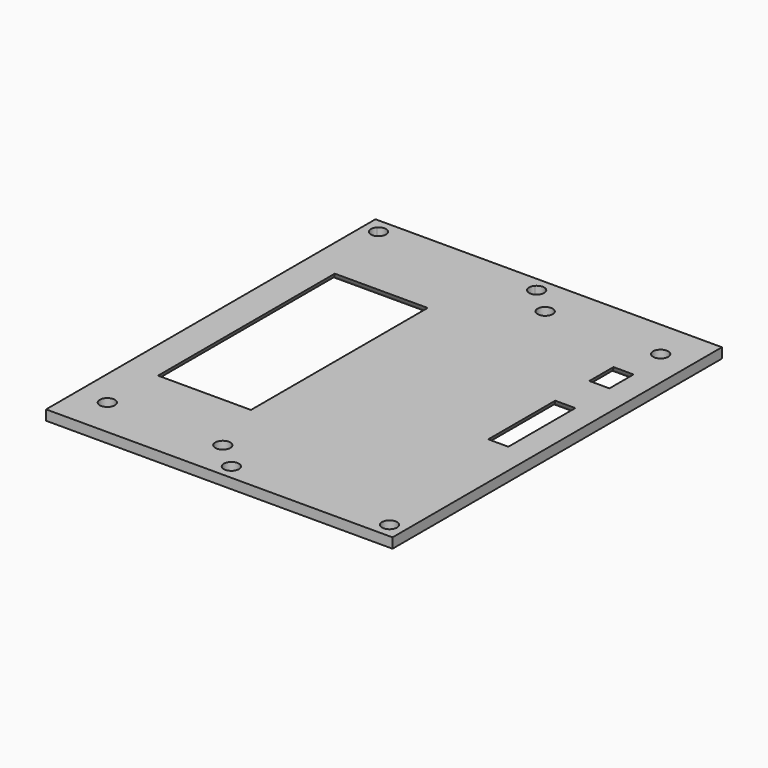
from build123d import *

# Parameters (mm, degrees)
F0_R          = 1.5
F0_W          = 18.5
F0_H          = 44
F0_W_2        = 4
F0_H_2        = 16.6644380502
F0_H_3        = 6
F0_W_3        = 4.7
F0_H_4        = 2
F0_W_4        = 13
F0_W_5        = 2.3
F0_W_6        = 1.5
F0_W_7        = 9
F0_W_8        = 11
F1_DEPTH      = 2
F2_T1_DEPTH   = 16.6644380502
F2_T3_DEPTH   = 4
F2_T5_DEPTH   = 6
F2_T7_DEPTH   = 44
F2_T9_DEPTH   = 18.5
F2_T15_DEPTH  = 11.0710678119
F2_T19_DEPTH  = 23.7355058621
F2_T26_DEPTH  = 11.0710678119
F2_T30_DEPTH  = 23.7355058621
F2_T37_DEPTH  = 23.7355058621
F2_T41_DEPTH  = 11.0710678119
F2_T49_DEPTH  = 11.0710678119
F2_T54_DEPTH  = 23.7355058621
F2_T61_DEPTH  = 13.0710678119
F2_T65_DEPTH  = 11.0710678119
F2_T73_DEPTH  = 13.0710678119
F2_T77_DEPTH  = 11.0710678119
F2_T84_DEPTH  = 11.0710678119
F2_T89_DEPTH  = 13.0710678119
F2_S91_R      = 1.5
F2_T92_DEPTH  = 8
F2_T98_DEPTH  = 13.0710678119
F2_T102_DEPTH = 11.0710678119
F2_T109_DEPTH = 25.5710678119
F2_T113_DEPTH = 51.0710678119
F2_T120_DEPTH = 51.0710678119
F2_T124_DEPTH = 25.5710678119
F2_T131_DEPTH = 51.0710678119
F2_T135_DEPTH = 25.5710678119
F2_T143_DEPTH = 51.0710678119
F2_T147_DEPTH = 25.5710678119


# Not quite as in the source:
# - a fillet or chamfer that OpenCascade refuses, or shapes differently, is made with other operations: its cross-section is extruded or revolved along the edge and cut away or added


with BuildPart() as f1:
    # F0 (on Top) → F1 (new body)
    with BuildSketch(Plane.XY):
        with BuildLine():
            Line((12.5, -41), (34.5, -41))
            Line((34.5, -41), (34.5, 39))
            Line((34.5, 39), (28.5, 39))
            Line((28.5, 39), (25.5, 39))
            Line((25.5, 39), (20.8, 39))
            Line((20.8, 39), (7.8, 39))
            Line((7.8, 39), (5.5, 39))
            Line((5.5, 39), (1.1180339887, 39))
            ThreePointArc((1.1180339887, 39), (1.4012585384, 38.5352331347), (1.5, 38))
            ThreePointArc((1.5, 38), (-0.5352331347, 36.5987414616), (-1.1180339887, 39))
            Line((-1.1180339887, 39), (-5.5, 39))
            Line((-5.5, 39), (-14.5, 39))
            Line((-14.5, 39), (-25.5, 39))
            Line((-25.5, 39), (-27, 39))
            Line((-27, 39), (-28.5, 39))
            Line((-28.5, 39), (-30.3819660113, 39))
            ThreePointArc((-30.3819660113, 39), (-30.0987414616, 38.5352331347), (-30, 38))
            ThreePointArc((-30, 38), (-32.0352331347, 36.5987414616), (-32.6180339887, 39))
            Line((-32.6180339887, 39), (-34.5, 39))
            Line((-34.5, 39), (-34.5, -41))
            Line((-34.5, -41), (-12.5, -41))
            Line((-12.5, -41), (-10.5, -41))
            Line((-10.5, -41), (10.5, -41))
            Line((10.5, -41), (12.5, -41))
        make_face()
        with Locations((-28.5, -33.25)):
            Circle(F0_R, mode=Mode.SUBTRACT)
        with Locations((-5.5, -33.25)):
            Circle(F0_R, mode=Mode.SUBTRACT)
        with Locations((0, -38)):
            Circle(F0_R, mode=Mode.SUBTRACT)
        with Locations((31.5, -38)):
            Circle(F0_R, mode=Mode.SUBTRACT)
        with Locations((-18.75, 0.75)):
            Rectangle(F0_W, F0_H, mode=Mode.SUBTRACT)
        with Locations((-28.5, 33.25)):
            Circle(F0_R, mode=Mode.SUBTRACT)
        with Locations((-5.5, 33.25)):
            Circle(F0_R, mode=Mode.SUBTRACT)
        with Locations((27.5, 2.4177809749)):
            Rectangle(F0_W_2, F0_H_2, mode=Mode.SUBTRACT)
        with Locations((5.5, 33.25)):
            Circle(F0_R, mode=Mode.SUBTRACT)
        with Locations((27.5, 22.25)):
            Rectangle(F0_W_2, F0_H_3, mode=Mode.SUBTRACT)
        with Locations((28.5, 33.25)):
            Circle(F0_R, mode=Mode.SUBTRACT)
        Polygon((28.5, 39), (34.5, 39), (34.5, 41), (28, 41), (25.5, 41), (25.5, 39), align=None)
        with Locations((23.15, 40)):
            Rectangle(F0_W_3, F0_H_4)
        with Locations((14.3, 40)):
            Rectangle(F0_W_4, F0_H_4)
        with Locations((6.65, 40)):
            Rectangle(F0_W_5, F0_H_4)
        with BuildLine():
            Line((-34.5, 41), (-34.5, 39))
            Line((-34.5, 39), (-32.6180339887, 39))
            ThreePointArc((-32.6180339887, 39), (-31.5, 39.5), (-30.3819660113, 39))
            Line((-30.3819660113, 39), (-28.5, 39))
            Line((-28.5, 39), (-27, 39))
            Line((-27, 39), (-27, 41))
            Line((-27, 41), (-34.5, 41))
        make_face()
        with BuildLine():
            Line((1.1180339887, 39), (5.5, 39))
            Line((5.5, 39), (5.5, 41))
            Line((5.5, 41), (-5.5, 41))
            Line((-5.5, 41), (-5.5, 39))
            Line((-5.5, 39), (-1.1180339887, 39))
            ThreePointArc((-1.1180339887, 39), (0, 39.5), (1.1180339887, 39))
        make_face()
        with Locations((-26.25, 40)):
            Rectangle(F0_W_6, F0_H_4)
        with Locations((-10, 40)):
            Rectangle(F0_W_7, F0_H_4)
        with Locations((-20, 40)):
            Rectangle(F0_W_8, F0_H_4)
        with Locations((-28.5, 33.25)):
            Circle(F0_R)
        with Locations((-5.5, 33.25)):
            Circle(F0_R)
    extrude(amount=F1_DEPTH)

    # F2: fillet of radius 3 on 12 edges, made by hand

    # F2_s2 → F2_t1 (cut)
    with BuildSketch(Plane.XZ.offset(-10.75)):
        with BuildLine():
            ThreePointArc((25.5, 2), (24.4036236828, 0.5505102572), (22.6715728753, 0))
            Line((22.6715728753, 0), (25.5, 0))
            Line((25.5, 0), (25.5, 2))
        make_face()
        with BuildLine():
            ThreePointArc((29.5, 2), (30.5963763172, 0.5505102572), (32.3284271247, 0))
            Line((32.3284271247, 0), (29.5, 0))
            Line((29.5, 0), (29.5, 2))
        make_face()
    extrude(amount=F2_T1_DEPTH, mode=Mode.SUBTRACT)

    # F2_s4 → F2_t3 (cut)
    with BuildSketch(Plane.YZ.offset(25.5)):
        with BuildLine():
            ThreePointArc((-5.9144380502, 2), (-7.0108143674, 0.5505102572), (-8.742865175, 0))
            Line((-8.742865175, 0), (-5.9144380502, 0))
            Line((-5.9144380502, 0), (-5.9144380502, 2))
        make_face()
        with BuildLine():
            ThreePointArc((10.75, 2), (11.8463763172, 0.5505102572), (13.5784271247, 0))
            Line((13.5784271247, 0), (10.75, 0))
            Line((10.75, 0), (10.75, 2))
        make_face()
        with BuildLine():
            ThreePointArc((19.25, 2), (18.1536236828, 0.5505102572), (16.4215728753, 0))
            Line((16.4215728753, 0), (19.25, 0))
            Line((19.25, 0), (19.25, 2))
        make_face()
        with BuildLine():
            ThreePointArc((25.25, 2), (26.3463763172, 0.5505102572), (28.0784271247, 0))
            Line((28.0784271247, 0), (25.25, 0))
            Line((25.25, 0), (25.25, 2))
        make_face()
    extrude(amount=F2_T3_DEPTH, mode=Mode.SUBTRACT)

    # F2_s6 → F2_t5 (cut)
    with BuildSketch(Plane.XZ.offset(-25.25)):
        with BuildLine():
            ThreePointArc((29.5, 2), (30.5963763172, 0.5505102572), (32.3284271247, 0))
            Line((32.3284271247, 0), (29.5, 0))
            Line((29.5, 0), (29.5, 2))
        make_face()
        with BuildLine():
            ThreePointArc((25.5, 2), (24.4036236828, 0.5505102572), (22.6715728753, 0))
            Line((22.6715728753, 0), (25.5, 0))
            Line((25.5, 0), (25.5, 2))
        make_face()
    extrude(amount=F2_T5_DEPTH, mode=Mode.SUBTRACT)

    # F2_s8 → F2_t7 (cut)
    with BuildSketch(Plane.XZ.offset(-22.75)):
        with BuildLine():
            ThreePointArc((-9.5, 2), (-8.4036236828, 0.5505102572), (-6.6715728753, 0))
            Line((-6.6715728753, 0), (-9.5, 0))
            Line((-9.5, 0), (-9.5, 2))
        make_face()
        with BuildLine():
            ThreePointArc((-28, 2), (-29.0963763172, 0.5505102572), (-30.8284271247, 0))
            Line((-30.8284271247, 0), (-28, 0))
            Line((-28, 0), (-28, 2))
        make_face()
    extrude(amount=F2_T7_DEPTH, mode=Mode.SUBTRACT)

    # F2_s10 → F2_t9 (cut)
    with BuildSketch(Plane.YZ.offset(-28)):
        with BuildLine():
            ThreePointArc((-21.25, 2), (-22.3463763172, 0.5505102572), (-24.0784271247, 0))
            Line((-24.0784271247, 0), (-21.25, 0))
            Line((-21.25, 0), (-21.25, 2))
        make_face()
        with BuildLine():
            ThreePointArc((22.75, 2), (23.8463763172, 0.5505102572), (25.5784271247, 0))
            Line((25.5784271247, 0), (22.75, 0))
            Line((22.75, 0), (22.75, 2))
        make_face()
    extrude(amount=F2_T9_DEPTH, mode=Mode.SUBTRACT)


with BuildPart() as f2_tool13:
    # F2_s14 → F2_t15 (new body)
    with BuildSketch(Plane.YZ.offset(29.5)):
        with BuildLine():
            ThreePointArc((-5.9144380502, 2), (-7.0108143674, 0.5505102572), (-8.742865175, 0))
            Line((-8.742865175, 0), (-5.9144380502, 0))
            Line((-5.9144380502, 0), (-5.9144380502, 2))
        make_face()
    extrude(amount=-F2_T15_DEPTH)

    split(bisect_by=Plane.YZ.offset(25.5), keep=Keep.BOTTOM)


with BuildPart() as f2_tool17:
    # F2_s18 → F2_t19 (new body)
    with BuildSketch(Plane.XZ.offset(12.9855058621)):
        with BuildLine():
            ThreePointArc((25.5, 2), (24.4036236828, 0.5505102572), (22.6715728753, 0))
            Line((22.6715728753, 0), (25.5, 0))
            Line((25.5, 0), (25.5, 2))
        make_face()
    extrude(amount=-F2_T19_DEPTH)

    split(bisect_by=Plane.XZ.offset(5.9144380502), keep=Keep.TOP)


with BuildPart() as f2_tool13_1:
    add(f2_tool13.part)

    # F2_t21: intersect F2_tool17
    add(f2_tool17.part, mode=Mode.INTERSECT)


with BuildPart() as f1_1:
    add(f1.part)

    # F2_t11: cut F2_tool13
    add(f2_tool13_1.part, mode=Mode.SUBTRACT)


with BuildPart() as f2_tool24:
    # F2_s25 → F2_t26 (new body)
    with BuildSketch(Plane.YZ.offset(18.4289321881)):
        with BuildLine():
            ThreePointArc((10.75, 2), (11.8463763172, 0.5505102572), (13.5784271247, 0))
            Line((13.5784271247, 0), (10.75, 0))
            Line((10.75, 0), (10.75, 2))
        make_face()
    extrude(amount=F2_T26_DEPTH)

    split(bisect_by=Plane.YZ.offset(25.5), keep=Keep.BOTTOM)


with BuildPart() as f2_tool28:
    # F2_s29 → F2_t30 (new body)
    with BuildSketch(Plane.XZ.offset(5.9144380502)):
        with BuildLine():
            ThreePointArc((25.5, 2), (24.4036236828, 0.5505102572), (22.6715728753, 0))
            Line((22.6715728753, 0), (25.5, 0))
            Line((25.5, 0), (25.5, 2))
        make_face()
    extrude(amount=-F2_T30_DEPTH)

    split(bisect_by=Plane.XZ.offset(-10.75), keep=Keep.BOTTOM)


with BuildPart() as f2_tool24_1:
    add(f2_tool24.part)

    # F2_t32: intersect F2_tool28
    add(f2_tool28.part, mode=Mode.INTERSECT)


with BuildPart() as f1_2:
    add(f1_1.part)

    # F2_t22: cut F2_tool24
    add(f2_tool24_1.part, mode=Mode.SUBTRACT)


with BuildPart() as f2_tool35:
    # F2_s36 → F2_t37 (new body)
    with BuildSketch(Plane.XZ.offset(-10.75)):
        with BuildLine():
            ThreePointArc((29.5, 2), (30.5963763172, 0.5505102572), (32.3284271247, 0))
            Line((32.3284271247, 0), (29.5, 0))
            Line((29.5, 0), (29.5, 2))
        make_face()
    extrude(amount=F2_T37_DEPTH)

    split(bisect_by=Plane.XZ.offset(5.9144380502), keep=Keep.TOP)


with BuildPart() as f2_tool39:
    # F2_s40 → F2_t41 (new body)
    with BuildSketch(Plane.YZ.offset(36.5710678119)):
        with BuildLine():
            ThreePointArc((-5.9144380502, 2), (-7.0108143674, 0.5505102572), (-8.742865175, 0))
            Line((-8.742865175, 0), (-5.9144380502, 0))
            Line((-5.9144380502, 0), (-5.9144380502, 2))
        make_face()
    extrude(amount=-F2_T41_DEPTH)

    split(bisect_by=Plane.YZ.offset(34.5), keep=Keep.BOTTOM)

    split(bisect_by=Plane.YZ.offset(29.5), keep=Keep.TOP)


with BuildPart() as f2_tool35_1:
    add(f2_tool35.part)

    # F2_t44: intersect F2_tool39
    add(f2_tool39.part, mode=Mode.INTERSECT)


with BuildPart() as f1_3:
    add(f1_2.part)

    # F2_t33: cut F2_tool35
    add(f2_tool35_1.part, mode=Mode.SUBTRACT)


with BuildPart() as f2_tool47:
    # F2_s48 → F2_t49 (new body)
    with BuildSketch(Plane.YZ.offset(25.5)):
        with BuildLine():
            ThreePointArc((10.75, 2), (11.8463763172, 0.5505102572), (13.5784271247, 0))
            Line((13.5784271247, 0), (10.75, 0))
            Line((10.75, 0), (10.75, 2))
        make_face()
    extrude(amount=F2_T49_DEPTH)

    split(bisect_by=Plane.YZ.offset(34.5), keep=Keep.BOTTOM)

    split(bisect_by=Plane.YZ.offset(29.5), keep=Keep.TOP)


with BuildPart() as f2_tool52:
    # F2_s53 → F2_t54 (new body)
    with BuildSketch(Plane.XZ.offset(-17.8210678119)):
        with BuildLine():
            ThreePointArc((29.5, 2), (30.5963763172, 0.5505102572), (32.3284271247, 0))
            Line((32.3284271247, 0), (29.5, 0))
            Line((29.5, 0), (29.5, 2))
        make_face()
    extrude(amount=F2_T54_DEPTH)

    split(bisect_by=Plane.XZ.offset(-10.75), keep=Keep.BOTTOM)


with BuildPart() as f2_tool47_1:
    add(f2_tool47.part)

    # F2_t56: intersect F2_tool52
    add(f2_tool52.part, mode=Mode.INTERSECT)


with BuildPart() as f1_4:
    add(f1_3.part)

    # F2_t45: cut F2_tool47
    add(f2_tool47_1.part, mode=Mode.SUBTRACT)


with BuildPart() as f2_tool59:
    # F2_s60 → F2_t61 (new body)
    with BuildSketch(Plane.XZ.offset(-25.25)):
        with BuildLine():
            ThreePointArc((29.5, 2), (30.5963763172, 0.5505102572), (32.3284271247, 0))
            Line((32.3284271247, 0), (29.5, 0))
            Line((29.5, 0), (29.5, 2))
        make_face()
    extrude(amount=F2_T61_DEPTH)

    split(bisect_by=Plane.XZ.offset(-19.25), keep=Keep.TOP)


with BuildPart() as f2_tool63:
    # F2_s64 → F2_t65 (new body)
    with BuildSketch(Plane.YZ.offset(36.5710678119)):
        with BuildLine():
            ThreePointArc((19.25, 2), (18.1536236828, 0.5505102572), (16.4215728753, 0))
            Line((16.4215728753, 0), (19.25, 0))
            Line((19.25, 0), (19.25, 2))
        make_face()
    extrude(amount=-F2_T65_DEPTH)

    split(bisect_by=Plane.YZ.offset(34.5), keep=Keep.BOTTOM)

    split(bisect_by=Plane.YZ.offset(29.5), keep=Keep.TOP)


with BuildPart() as f2_tool59_1:
    add(f2_tool59.part)

    # F2_t68: intersect F2_tool63
    add(f2_tool63.part, mode=Mode.INTERSECT)


with BuildPart() as f1_5:
    add(f1_4.part)

    # F2_t57: cut F2_tool59
    add(f2_tool59_1.part, mode=Mode.SUBTRACT)


with BuildPart() as f2_tool71:
    # F2_s72 → F2_t73 (new body)
    with BuildSketch(Plane.XZ.offset(-12.1789321881)):
        with BuildLine():
            ThreePointArc((25.5, 2), (24.4036236828, 0.5505102572), (22.6715728753, 0))
            Line((22.6715728753, 0), (25.5, 0))
            Line((25.5, 0), (25.5, 2))
        make_face()
    extrude(amount=-F2_T73_DEPTH)

    split(bisect_by=Plane.XZ.offset(-19.25), keep=Keep.TOP)


with BuildPart() as f2_tool75:
    # F2_s76 → F2_t77 (new body)
    with BuildSketch(Plane.YZ.offset(29.5)):
        with BuildLine():
            ThreePointArc((19.25, 2), (18.1536236828, 0.5505102572), (16.4215728753, 0))
            Line((16.4215728753, 0), (19.25, 0))
            Line((19.25, 0), (19.25, 2))
        make_face()
    extrude(amount=-F2_T77_DEPTH)

    split(bisect_by=Plane.YZ.offset(25.5), keep=Keep.BOTTOM)


with BuildPart() as f2_tool71_1:
    add(f2_tool71.part)

    # F2_t79: intersect F2_tool75
    add(f2_tool75.part, mode=Mode.INTERSECT)


with BuildPart() as f1_6:
    add(f1_5.part)

    # F2_t69: cut F2_tool71
    add(f2_tool71_1.part, mode=Mode.SUBTRACT)


with BuildPart() as f2_tool82:
    # F2_s83 → F2_t84 (new body)
    with BuildSketch(Plane.YZ.offset(25.5)):
        with BuildLine():
            ThreePointArc((25.25, 2), (26.3463763172, 0.5505102572), (28.0784271247, 0))
            Line((28.0784271247, 0), (25.25, 0))
            Line((25.25, 0), (25.25, 2))
        make_face()
    extrude(amount=F2_T84_DEPTH)

    split(bisect_by=Plane.YZ.offset(34.5), keep=Keep.BOTTOM)

    split(bisect_by=Plane.YZ.offset(29.5), keep=Keep.TOP)


with BuildPart() as f2_tool87:
    # F2_s88 → F2_t89 (new body)
    with BuildSketch(Plane.XZ.offset(-32.3210678119)):
        with BuildLine():
            ThreePointArc((29.5, 2), (30.5963763172, 0.5505102572), (32.3284271247, 0))
            Line((32.3284271247, 0), (29.5, 0))
            Line((29.5, 0), (29.5, 2))
        make_face()
    extrude(amount=F2_T89_DEPTH)

    split(bisect_by=Plane.XZ.offset(-25.25), keep=Keep.BOTTOM)

    # F2_s91 → F2_t92 (cut, symmetric)
    with BuildSketch(Plane.XY.offset(1)):
        with Locations((28.5, 33.25)):
            Circle(F2_S91_R)
    extrude(amount=F2_T92_DEPTH, both=True, mode=Mode.SUBTRACT)


with BuildPart() as f2_tool82_1:
    add(f2_tool82.part)

    # F2_t93: intersect F2_tool87
    add(f2_tool87.part, mode=Mode.INTERSECT)


with BuildPart() as f1_7:
    add(f1_6.part)

    # F2_t80: cut F2_tool82
    add(f2_tool82_1.part, mode=Mode.SUBTRACT)


with BuildPart() as f2_tool96:
    # F2_s97 → F2_t98 (new body)
    with BuildSketch(Plane.XZ.offset(-19.25)):
        with BuildLine():
            ThreePointArc((25.5, 2), (24.4036236828, 0.5505102572), (22.6715728753, 0))
            Line((22.6715728753, 0), (25.5, 0))
            Line((25.5, 0), (25.5, 2))
        make_face()
    extrude(amount=-F2_T98_DEPTH)

    split(bisect_by=Plane.XZ.offset(-25.25), keep=Keep.BOTTOM)


with BuildPart() as f2_tool100:
    # F2_s101 → F2_t102 (new body)
    with BuildSketch(Plane.YZ.offset(18.4289321881)):
        with BuildLine():
            ThreePointArc((25.25, 2), (26.3463763172, 0.5505102572), (28.0784271247, 0))
            Line((28.0784271247, 0), (25.25, 0))
            Line((25.25, 0), (25.25, 2))
        make_face()
    extrude(amount=F2_T102_DEPTH)

    split(bisect_by=Plane.YZ.offset(25.5), keep=Keep.BOTTOM)


with BuildPart() as f2_tool96_1:
    add(f2_tool96.part)

    # F2_t104: intersect F2_tool100
    add(f2_tool100.part, mode=Mode.INTERSECT)


with BuildPart() as f1_8:
    add(f1_7.part)

    # F2_t94: cut F2_tool96
    add(f2_tool96_1.part, mode=Mode.SUBTRACT)


with BuildPart() as f2_tool107:
    # F2_s108 → F2_t109 (new body)
    with BuildSketch(Plane.YZ.offset(-28)):
        with BuildLine():
            ThreePointArc((22.75, 2), (23.8463763172, 0.5505102572), (25.5784271247, 0))
            Line((25.5784271247, 0), (22.75, 0))
            Line((22.75, 0), (22.75, 2))
        make_face()
    extrude(amount=F2_T109_DEPTH)

    split(bisect_by=Plane.YZ.offset(-9.5), keep=Keep.TOP)


with BuildPart() as f2_tool111:
    # F2_s112 → F2_t113 (new body)
    with BuildSketch(Plane.XZ.offset(-29.8210678119)):
        with BuildLine():
            ThreePointArc((-9.5, 2), (-8.4036236828, 0.5505102572), (-6.6715728753, 0))
            Line((-6.6715728753, 0), (-9.5, 0))
            Line((-9.5, 0), (-9.5, 2))
        make_face()
    extrude(amount=F2_T113_DEPTH)

    split(bisect_by=Plane.XZ.offset(-22.75), keep=Keep.BOTTOM)


with BuildPart() as f2_tool107_1:
    add(f2_tool107.part)

    # F2_t115: intersect F2_tool111
    add(f2_tool111.part, mode=Mode.INTERSECT)


with BuildPart() as f1_9:
    add(f1_8.part)

    # F2_t105: cut F2_tool107
    add(f2_tool107_1.part, mode=Mode.SUBTRACT)


with BuildPart() as f2_tool118:
    # F2_s119 → F2_t120 (new body)
    with BuildSketch(Plane.XZ.offset(-22.75)):
        with BuildLine():
            ThreePointArc((-9.5, 2), (-8.4036236828, 0.5505102572), (-6.6715728753, 0))
            Line((-6.6715728753, 0), (-9.5, 0))
            Line((-9.5, 0), (-9.5, 2))
        make_face()
    extrude(amount=F2_T120_DEPTH)

    split(bisect_by=Plane.XZ.offset(21.25), keep=Keep.TOP)


with BuildPart() as f2_tool122:
    # F2_s123 → F2_t124 (new body)
    with BuildSketch(Plane.YZ.offset(-2.4289321881)):
        with BuildLine():
            ThreePointArc((-21.25, 2), (-22.3463763172, 0.5505102572), (-24.0784271247, 0))
            Line((-24.0784271247, 0), (-21.25, 0))
            Line((-21.25, 0), (-21.25, 2))
        make_face()
    extrude(amount=-F2_T124_DEPTH)

    split(bisect_by=Plane.YZ.offset(-9.5), keep=Keep.TOP)


with BuildPart() as f2_tool118_1:
    add(f2_tool118.part)

    # F2_t126: intersect F2_tool122
    add(f2_tool122.part, mode=Mode.INTERSECT)


with BuildPart() as f1_10:
    add(f1_9.part)

    # F2_t116: cut F2_tool118
    add(f2_tool118_1.part, mode=Mode.SUBTRACT)


with BuildPart() as f2_tool129:
    # F2_s130 → F2_t131 (new body)
    with BuildSketch(Plane.XZ.offset(28.3210678119)):
        with BuildLine():
            ThreePointArc((-28, 2), (-29.0963763172, 0.5505102572), (-30.8284271247, 0))
            Line((-30.8284271247, 0), (-28, 0))
            Line((-28, 0), (-28, 2))
        make_face()
    extrude(amount=-F2_T131_DEPTH)

    split(bisect_by=Plane.XZ.offset(21.25), keep=Keep.TOP)


with BuildPart() as f2_tool133:
    # F2_s134 → F2_t135 (new body)
    with BuildSketch(Plane.YZ.offset(-9.5)):
        with BuildLine():
            ThreePointArc((-21.25, 2), (-22.3463763172, 0.5505102572), (-24.0784271247, 0))
            Line((-24.0784271247, 0), (-21.25, 0))
            Line((-21.25, 0), (-21.25, 2))
        make_face()
    extrude(amount=-F2_T135_DEPTH)

    split(bisect_by=Plane.YZ.offset(-34.5), keep=Keep.TOP)

    split(bisect_by=Plane.YZ.offset(-28), keep=Keep.BOTTOM)


with BuildPart() as f2_tool129_1:
    add(f2_tool129.part)

    # F2_t138: intersect F2_tool133
    add(f2_tool133.part, mode=Mode.INTERSECT)


with BuildPart() as f1_11:
    add(f1_10.part)

    # F2_t127: cut F2_tool129
    add(f2_tool129_1.part, mode=Mode.SUBTRACT)


with BuildPart() as f2_tool141:
    # F2_s142 → F2_t143 (new body)
    with BuildSketch(Plane.XZ.offset(21.25)):
        with BuildLine():
            ThreePointArc((-28, 2), (-29.0963763172, 0.5505102572), (-30.8284271247, 0))
            Line((-30.8284271247, 0), (-28, 0))
            Line((-28, 0), (-28, 2))
        make_face()
    extrude(amount=-F2_T143_DEPTH)

    split(bisect_by=Plane.XZ.offset(-22.75), keep=Keep.BOTTOM)


with BuildPart() as f2_tool145:
    # F2_s146 → F2_t147 (new body)
    with BuildSketch(Plane.YZ.offset(-35.0710678119)):
        with BuildLine():
            ThreePointArc((22.75, 2), (23.8463763172, 0.5505102572), (25.5784271247, 0))
            Line((25.5784271247, 0), (22.75, 0))
            Line((22.75, 0), (22.75, 2))
        make_face()
    extrude(amount=F2_T147_DEPTH)

    split(bisect_by=Plane.YZ.offset(-34.5), keep=Keep.TOP)

    split(bisect_by=Plane.YZ.offset(-28), keep=Keep.BOTTOM)


with BuildPart() as f2_tool141_1:
    add(f2_tool141.part)

    # F2_t150: intersect F2_tool145
    add(f2_tool145.part, mode=Mode.INTERSECT)


with BuildPart() as f1_12:
    add(f1_11.part)

    # F2_t139: cut F2_tool141
    add(f2_tool141_1.part, mode=Mode.SUBTRACT)


solid = f1_12.part
